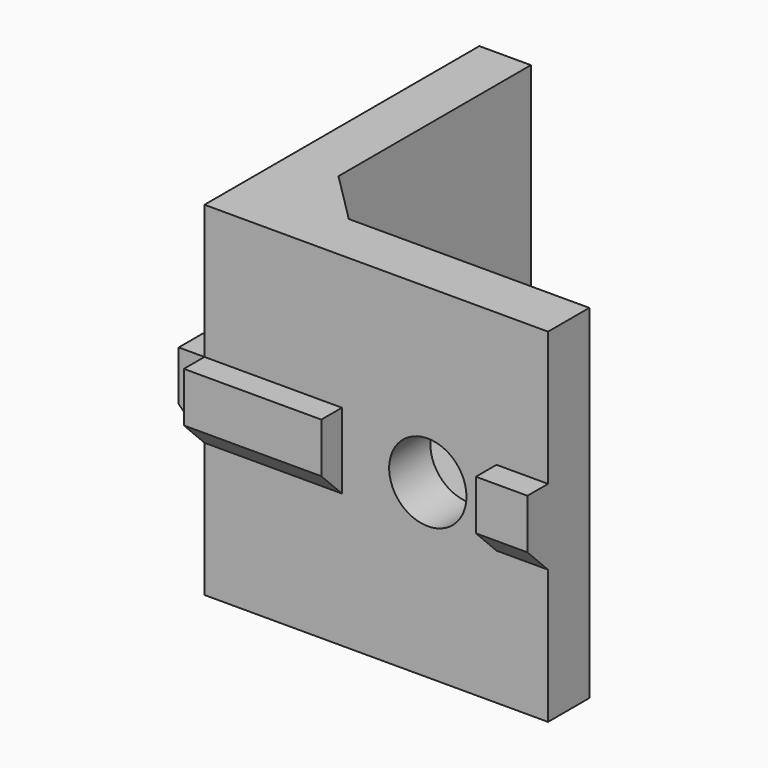
from build123d import *

# Parameters (mm, degrees)
F1_DEPTH = 20
F2_DEPTH = 4
F3_R     = 2.25
F4_DEPTH = 3
F3_W     = 8
F3_H     = 4.4
F3_W_2   = 3
F5_DEPTH = 1.5
F6_SIZE  = 1.49999
F8_SIZE  = 3


# Not quite as in the source:
# - a fillet or chamfer is up to 0.001 mm smaller than in the source, because OpenCascade refuses the exact size
# - a pattern or mirror of a feature is missing from the dataset's text; its kind, count and spacing are read off the source's solid


with BuildPart() as f1:
    # F0 (on Top) → F1 (new body)
    with BuildSketch(Plane.XY):
        Polygon((0, 20), (0, 0), (20, 0), (20, 3), (3, 3), (3, 20), align=None)
    extrude(amount=F1_DEPTH)

    # F0 (on Top) → F2 (join)
    with BuildSketch(Plane.XY):
        Polygon((3, 3), (20, 3), (3, 20), align=None)
    extrude(amount=F2_DEPTH)

    # F3 (on face) → F4 (cut, through all)
    with BuildSketch(Plane.XZ):
        with Locations((13, 10)):
            Circle(F3_R)
    f4 = extrude(amount=-F4_DEPTH, mode=Mode.SUBTRACT)

    # F4_copies: F4 across plane
    add(f4.mirror(Plane(origin=(0, 0, 0), x_dir=(-0.7071067812, -0.7071067812, 0), z_dir=(-0.7071067812, 0.7071067812, 0))), mode=Mode.SUBTRACT)

    # F3 (on face) → F5 (join)
    with BuildSketch(Plane.XZ):
        with Locations((4, 10)):
            Rectangle(F3_W, F3_H)
        with Locations((18.5, 10)):
            Rectangle(F3_W_2, F3_H)
    f5 = extrude(amount=F5_DEPTH)

    # F5_copies: F5 across plane
    add(f5.mirror(Plane(origin=(0, 0, 0), x_dir=(0.7071067812, 0.7071067812, 0), z_dir=(-0.7071067812, 0.7071067812, 0))))

    # F6 (size 1.5 in the source; OpenCascade refuses exactly that, so slightly less here)
    f6_edges = [f1.edges().sort_by_distance(p)[0] for p in [
        (4, -1.5, 7.8),
        (18.5, -1.5, 7.8),
        (-1.5, 4, 7.8),
        (-1.5, 18.5, 7.8),
    ]]
    chamfer(f6_edges, length=F6_SIZE)

    # F8
    f8_edges = [f1.edges().sort_by_distance(p)[0] for p in [
        (3, 3, 12),
    ]]
    chamfer(f8_edges, length=F8_SIZE)


solid = f1.part
